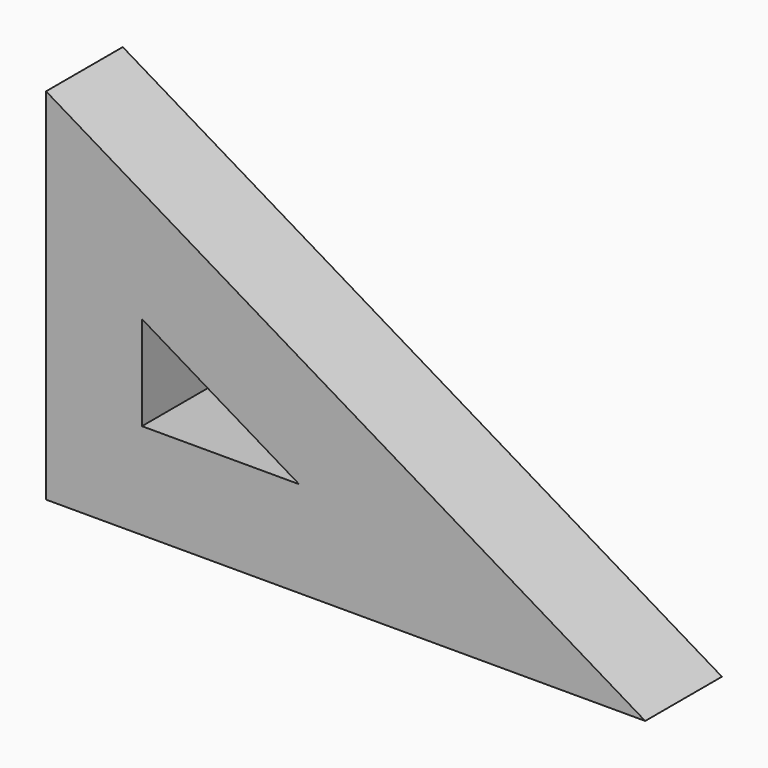
from build123d import *

# Parameters (mm, degrees)
F1_DEPTH = 40


# Not quite as in the source:
# - a feature names something its author has since deleted; it is built from what else it names


with BuildPart() as f1:
    # F0 (on Front) → F1 (new body)
    with BuildSketch(Plane.XZ):
        Polygon((0, 150), (0, 0), (250, 0), align=None)
        Polygon((105.5873080687, 40), (40, 40), (40, 79.3523848412), align=None, mode=Mode.SUBTRACT)
    extrude(amount=F1_DEPTH)


solid = f1.part
